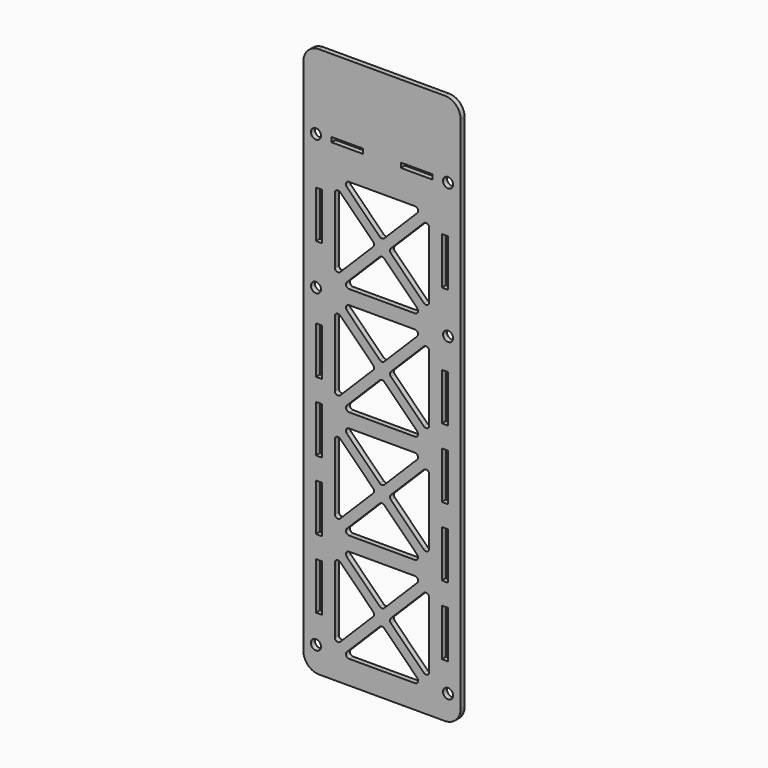
from build123d import *

# Parameters (mm, degrees)
F0_R     = 1.6
F0_W     = 2
F0_H     = 15
F0_W_2   = 10
F0_H_2   = 1.5
F1_DEPTH = 1.5875


# Not quite as in the source:
# - ends of sketch curves that miss each other by under 0.0002 mm in the source are joined


with BuildPart() as f1:
    # F0 (on Front) → F1 (new body)
    with BuildSketch(Plane.XZ):
        with BuildLine():
            Line((25, -82.5), (25, 82.5))
            ThreePointArc((25, 82.5), (23.5355339059, 86.0355339059), (20, 87.5))
            Line((20, 87.5), (-20, 87.5))
            ThreePointArc((-20, 87.5), (-23.5355339059, 86.0355339059), (-25, 82.5))
            Line((-25, 82.5), (-25, -82.5))
            ThreePointArc((-25, -82.5), (-23.5355339059, -86.0355339059), (-20, -87.5))
            Line((-20, -87.5), (20, -87.5))
            ThreePointArc((20, -87.5), (23.5355339059, -86.0355339059), (25, -82.5))
        make_face()
        with Locations((-21, -79.5)):
            Circle(F0_R, mode=Mode.SUBTRACT)
        with Locations((-20, -63)):
            Rectangle(F0_W, F0_H, mode=Mode.SUBTRACT)
        with BuildLine():
            ThreePointArc((-0.7071067812, -67.8284272188), (0, -67.535534), (0.7071067812, -67.8284272188))
            Line((0.7071067812, -67.8284272188), (11.171573, -78.292893))
            ThreePointArc((11.171573, -78.292893), (11.3883455325, -79.3826834324), (10.464466, -80))
            Line((10.464466, -80), (-10.464466, -80))
            ThreePointArc((-10.464466, -80), (-11.3883455325, -79.3826834324), (-11.1715727812, -78.2928932188))
            Line((-11.1715727812, -78.2928932188), (-0.7071067812, -67.8284272188))
        make_face(mode=Mode.SUBTRACT)
        with BuildLine():
            ThreePointArc((-15, -54.535534), (-14.3826834324, -53.6116544675), (-13.2928932188, -53.8284272188))
            Line((-13.2928932188, -53.8284272188), (-2.828427, -64.292893))
            ThreePointArc((-2.828427, -64.292893), (-2.535534, -65), (-2.8284272188, -65.7071067812))
            Line((-2.8284272188, -65.7071067812), (-13.292893, -76.171573))
            ThreePointArc((-13.292893, -76.171573), (-14.3826834324, -76.3883455325), (-15, -75.464466))
            Line((-15, -75.464466), (-15, -54.535534))
        make_face(mode=Mode.SUBTRACT)
        with Locations((-20, -41)):
            Rectangle(F0_W, F0_H, mode=Mode.SUBTRACT)
        with Locations((-20, -19)):
            Rectangle(F0_W, F0_H, mode=Mode.SUBTRACT)
        with BuildLine():
            ThreePointArc((-15, -20.035534), (-14.3826834324, -19.1116544675), (-13.2928932188, -19.3284272188))
            Line((-13.2928932188, -19.3284272188), (-2.828427, -29.792893))
            ThreePointArc((-2.828427, -29.792893), (-2.535534, -30.5), (-2.8284272188, -31.2071067812))
            Line((-2.8284272188, -31.2071067812), (-13.292893, -41.671573))
            ThreePointArc((-13.292893, -41.671573), (-14.3826834324, -41.8883455325), (-15, -40.964466))
            Line((-15, -40.964466), (-15, -20.035534))
        make_face(mode=Mode.SUBTRACT)
        with BuildLine():
            ThreePointArc((0.7071067812, -62.1715727812), (0, -62.464466), (-0.7071067812, -62.1715727812))
            Line((-0.7071067812, -62.1715727812), (-11.171573, -51.707107))
            ThreePointArc((-11.171573, -51.707107), (-11.3883455325, -50.6173165676), (-10.464466, -50))
            Line((-10.464466, -50), (10.464466, -50))
            ThreePointArc((10.464466, -50), (11.3883455325, -50.6173165676), (11.1715727812, -51.7071067812))
            Line((11.1715727812, -51.7071067812), (0.7071067812, -62.1715727812))
        make_face(mode=Mode.SUBTRACT)
        with BuildLine():
            ThreePointArc((13.2928932188, -53.8284272188), (14.3826834324, -53.6116544675), (15, -54.535534))
            Line((15, -54.535534), (15, -75.464466))
            ThreePointArc((15, -75.464466), (14.3826834324, -76.3883455325), (13.2928932188, -76.1715727812))
            Line((13.2928932188, -76.1715727812), (2.828427, -65.707107))
            ThreePointArc((2.828427, -65.707107), (2.535534, -65), (2.8284272188, -64.2928932188))
            Line((2.8284272188, -64.2928932188), (13.2928932188, -53.8284272188))
        make_face(mode=Mode.SUBTRACT)
        with Locations((21, -79.5)):
            Circle(F0_R, mode=Mode.SUBTRACT)
        with Locations((20, -63)):
            Rectangle(F0_W, F0_H, mode=Mode.SUBTRACT)
        with BuildLine():
            ThreePointArc((-0.7071067812, -33.3284272188), (0, -33.035534), (0.7071067812, -33.3284272188))
            Line((0.7071067812, -33.3284272188), (11.171573, -43.792893))
            ThreePointArc((11.171573, -43.792893), (11.3883455325, -44.8826834324), (10.464466, -45.5))
            Line((10.464466, -45.5), (-10.464466, -45.5))
            ThreePointArc((-10.464466, -45.5), (-11.3883455325, -44.8826834324), (-11.1715727812, -43.7928932188))
            Line((-11.1715727812, -43.7928932188), (-0.7071067812, -33.3284272188))
        make_face(mode=Mode.SUBTRACT)
        with BuildLine():
            ThreePointArc((13.2928932188, -19.3284272188), (14.3826834324, -19.1116544675), (15, -20.035534))
            Line((15, -20.035534), (15, -40.964466))
            ThreePointArc((15, -40.964466), (14.3826834324, -41.8883455325), (13.2928932188, -41.6715727812))
            Line((13.2928932188, -41.6715727812), (2.828427, -31.207107))
            ThreePointArc((2.828427, -31.207107), (2.535534, -30.5), (2.8284272188, -29.7928932188))
            Line((2.8284272188, -29.7928932188), (13.2928932188, -19.3284272188))
        make_face(mode=Mode.SUBTRACT)
        with BuildLine():
            ThreePointArc((0.7071067812, -27.6715727812), (0, -27.964466), (-0.7071067812, -27.6715727812))
            Line((-0.7071067812, -27.6715727812), (-11.171573, -17.207107))
            ThreePointArc((-11.171573, -17.207107), (-11.3883455325, -16.1173165676), (-10.464466, -15.5))
            Line((-10.464466, -15.5), (10.464466, -15.5))
            ThreePointArc((10.464466, -15.5), (11.3883455325, -16.1173165676), (11.1715727812, -17.2071067812))
            Line((11.1715727812, -17.2071067812), (0.7071067812, -27.6715727812))
        make_face(mode=Mode.SUBTRACT)
        with BuildLine():
            ThreePointArc((-0.7071067812, 1.1715727812), (0, 1.464466), (0.7071067812, 1.1715727812))
            Line((0.7071067812, 1.1715727812), (11.171573, -9.292893))
            ThreePointArc((11.171573, -9.292893), (11.3883455325, -10.3826834324), (10.464466, -11))
            Line((10.464466, -11), (-10.464466, -11))
            ThreePointArc((-10.464466, -11), (-11.3883455325, -10.3826834324), (-11.1715727812, -9.2928932188))
            Line((-11.1715727812, -9.2928932188), (-0.7071067812, 1.1715727812))
        make_face(mode=Mode.SUBTRACT)
        with Locations((20, -41)):
            Rectangle(F0_W, F0_H, mode=Mode.SUBTRACT)
        with Locations((20, -19)):
            Rectangle(F0_W, F0_H, mode=Mode.SUBTRACT)
        with Locations((-20, 3)):
            Rectangle(F0_W, F0_H, mode=Mode.SUBTRACT)
        with Locations((-21, 20.5)):
            Circle(F0_R, mode=Mode.SUBTRACT)
        with Locations((-20, 41)):
            Rectangle(F0_W, F0_H, mode=Mode.SUBTRACT)
        with BuildLine():
            ThreePointArc((-15, 14.464466), (-14.3826834324, 15.3883455325), (-13.2928932188, 15.1715727812))
            Line((-13.2928932188, 15.1715727812), (-2.828427, 4.707107))
            ThreePointArc((-2.828427, 4.707107), (-2.535534, 4), (-2.8284272188, 3.2928932188))
            Line((-2.8284272188, 3.2928932188), (-13.292893, -7.171573))
            ThreePointArc((-13.292893, -7.171573), (-14.3826834324, -7.3883455325), (-15, -6.464466))
            Line((-15, -6.464466), (-15, 14.464466))
        make_face(mode=Mode.SUBTRACT)
        with BuildLine():
            ThreePointArc((-15, 48.964466), (-14.3826834324, 49.8883455325), (-13.2928932188, 49.6715727812))
            Line((-13.2928932188, 49.6715727812), (-2.828427, 39.207107))
            ThreePointArc((-2.828427, 39.207107), (-2.535534, 38.5), (-2.8284272188, 37.7928932188))
            Line((-2.8284272188, 37.7928932188), (-13.292893, 27.328427))
            ThreePointArc((-13.292893, 27.328427), (-14.3826834324, 27.1116544675), (-15, 28.035534))
            Line((-15, 28.035534), (-15, 48.964466))
        make_face(mode=Mode.SUBTRACT)
        with Locations((-21, 63.5)):
            Circle(F0_R, mode=Mode.SUBTRACT)
        with Locations((-11, 63.5)):
            Rectangle(F0_W_2, F0_H_2, mode=Mode.SUBTRACT)
        with BuildLine():
            ThreePointArc((0.7071067812, 6.8284272188), (0, 6.535534), (-0.7071067812, 6.8284272188))
            Line((-0.7071067812, 6.8284272188), (-11.171573, 17.292893))
            ThreePointArc((-11.171573, 17.292893), (-11.3883455325, 18.3826834324), (-10.464466, 19))
            Line((-10.464466, 19), (10.464466, 19))
            ThreePointArc((10.464466, 19), (11.3883455325, 18.3826834324), (11.1715727812, 17.2928932188))
            Line((11.1715727812, 17.2928932188), (0.7071067812, 6.8284272188))
        make_face(mode=Mode.SUBTRACT)
        with BuildLine():
            ThreePointArc((13.2928932188, 15.1715727812), (14.3826834324, 15.3883455325), (15, 14.464466))
            Line((15, 14.464466), (15, -6.464466))
            ThreePointArc((15, -6.464466), (14.3826834324, -7.3883455325), (13.2928932188, -7.1715727812))
            Line((13.2928932188, -7.1715727812), (2.828427, 3.292893))
            ThreePointArc((2.828427, 3.292893), (2.535534, 4), (2.8284272188, 4.7071067812))
            Line((2.8284272188, 4.7071067812), (13.2928932188, 15.1715727812))
        make_face(mode=Mode.SUBTRACT)
        with BuildLine():
            ThreePointArc((-0.7071067812, 35.6715727812), (0, 35.964466), (0.7071067812, 35.6715727812))
            Line((0.7071067812, 35.6715727812), (11.171573, 25.207107))
            ThreePointArc((11.171573, 25.207107), (11.3883455325, 24.1173165676), (10.464466, 23.5))
            Line((10.464466, 23.5), (-10.464466, 23.5))
            ThreePointArc((-10.464466, 23.5), (-11.3883455325, 24.1173165676), (-11.1715727812, 25.2071067812))
            Line((-11.1715727812, 25.2071067812), (-0.7071067812, 35.6715727812))
        make_face(mode=Mode.SUBTRACT)
        with BuildLine():
            ThreePointArc((13.2928932188, 49.6715727812), (14.3826834324, 49.8883455325), (15, 48.964466))
            Line((15, 48.964466), (15, 28.035534))
            ThreePointArc((15, 28.035534), (14.3826834324, 27.1116544675), (13.2928932188, 27.3284272188))
            Line((13.2928932188, 27.3284272188), (2.828427, 37.792893))
            ThreePointArc((2.828427, 37.792893), (2.535534, 38.5), (2.8284272188, 39.2071067812))
            Line((2.8284272188, 39.2071067812), (13.2928932188, 49.6715727812))
        make_face(mode=Mode.SUBTRACT)
        with Locations((20, 3)):
            Rectangle(F0_W, F0_H, mode=Mode.SUBTRACT)
        with Locations((21, 20.5)):
            Circle(F0_R, mode=Mode.SUBTRACT)
        with Locations((20, 41)):
            Rectangle(F0_W, F0_H, mode=Mode.SUBTRACT)
        with BuildLine():
            ThreePointArc((0.7071067812, 41.3284272188), (0, 41.035534), (-0.7071067812, 41.3284272188))
            Line((-0.7071067812, 41.3284272188), (-11.171573, 51.792893))
            ThreePointArc((-11.171573, 51.792893), (-11.3883455325, 52.8826834324), (-10.464466, 53.5))
            Line((-10.464466, 53.5), (10.464466, 53.5))
            ThreePointArc((10.464466, 53.5), (11.3883455325, 52.8826834324), (11.1715727812, 51.7928932188))
            Line((11.1715727812, 51.7928932188), (0.7071067812, 41.3284272188))
        make_face(mode=Mode.SUBTRACT)
        with Locations((11, 63.5)):
            Rectangle(F0_W_2, F0_H_2, mode=Mode.SUBTRACT)
        with Locations((21, 63.5)):
            Circle(F0_R, mode=Mode.SUBTRACT)
    extrude(amount=F1_DEPTH)


solid = f1.part
